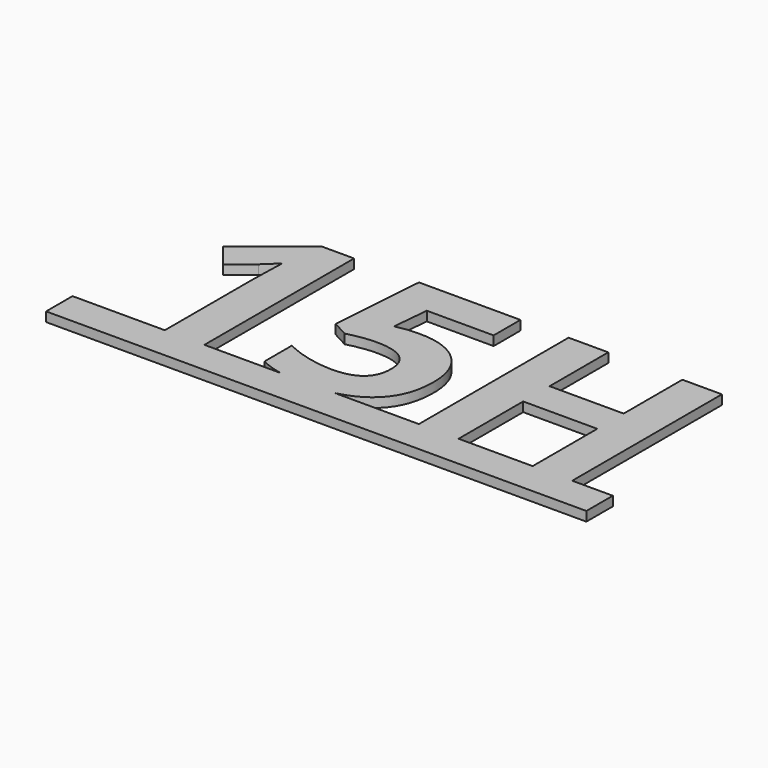
from build123d import *

# Parameters (mm, degrees)
F1_DEPTH = 50.8


# Not quite as in the source:
# - a feature names something its author has since deleted; it is built from what else it names


with BuildPart() as f1:
    # F0 (on Top) → F1 (new body)
    with BuildSketch(Plane.XY):
        with BuildLine():
            Line((-283.7137092352, 0), (-283.7137092352, -177.8))
            Line((-283.7137092352, -177.8), (2624.9390685426, -177.8))
            Line((2624.9390685426, -177.8), (2624.9390685426, 0))
            Line((2624.9390685426, 0), (2406.4373324315, 0))
            Line((2406.4373324315, 0), (2193.4477490981, 0))
            Line((2193.4477490981, 0), (1794.5883740981, 0))
            Line((1794.5883740981, 0), (1580.9373324315, 0))
            Line((1580.9373324315, 0), (1126.7145519045, 0))
            add(Edge.make_bspline(
                [(1126.7145519045, 0), (1064.7611763958, -13.890625), (989.1526102093, -13.890625)],
                knots=[0.6094332671, 0.6094332671, 0.6094332671, 1, 1, 1], degree=2))
            add(Edge.make_bspline(
                [(989.1526102093, -13.890625), (904.1900533476, -13.890625), (835.8175141984, 0)],
                knots=[0, 0, 0, 0.5050353738, 0.5050353738, 0.5050353738], degree=2))
            Line((835.8175141984, 0), (426.2515685426, 0))
            Line((426.2515685426, 0), (213.2619852093, 0))
            Line((213.2619852093, 0), (-283.7137092352, 0))
        make_face()
        with BuildLine():
            add(Edge.make_bspline(
                [(835.8175141984, 0), (768.808369802, 13.6136365267), (717.7342074315, 40.5694444444)],
                knots=[0.5050353738, 0.5050353738, 0.5050353738, 1, 1, 1], degree=2))
            Line((835.8175141984, 0), (1126.7145519045, 0))
            add(Edge.make_bspline(
                [(1286.8088602093, 77.1701388889), (1223.3854786806, 21.6746800513), (1126.7145519045, 0)],
                knots=[0, 0, 0, 0.6094332671, 0.6094332671, 0.6094332671], degree=2))
            add(Edge.make_bspline(
                [(1390.8783046537, 336.9027777778), (1390.8783046537, 168.2309027778), (1286.8088602093, 77.1701388889)],
                knots=[0, 0, 0, 1, 1, 1], degree=2))
            add(Edge.make_bspline(
                [(1304.3375060426, 561.578125), (1390.8783046537, 479.5572916667), (1390.8783046537, 336.9027777778)],
                knots=[0, 0, 0, 1, 1, 1], degree=2))
            add(Edge.make_bspline(
                [(1071.8349018759, 643.5989583333), (1217.7967074315, 643.5989583333), (1304.3375060426, 561.578125)],
                knots=[0, 0, 0, 1, 1, 1], degree=2))
            add(Edge.make_bspline(
                [(967.7654574315, 633.8975694444), (1009.8783046537, 643.5989583333), (1071.8349018759, 643.5989583333)],
                knots=[0, 0, 0, 1, 1, 1], degree=2))
            Line((967.7654574315, 633.8975694444), (943.7324713204, 629.046875))
            Line((943.7324713204, 629.046875), (962.2533046537, 826.8229166667))
            Line((962.2533046537, 826.8229166667), (1321.8661518759, 826.8229166667))
            Line((1321.8661518759, 826.8229166667), (1321.8661518759, 1007.4010416667))
            Line((1321.8661518759, 1007.4010416667), (775.5015685426, 1007.4010416667))
            Line((775.5015685426, 1007.4010416667), (737.5779574315, 494.109375))
            Line((737.5779574315, 494.109375), (822.4651102093, 448.46875))
            add(Edge.make_bspline(
                [(894.1230963204, 464.1232638889), (850.0258740981, 456.8472222222), (822.4651102093, 448.46875)],
                knots=[0, 0, 0, 1, 1, 1], degree=2))
            add(Edge.make_bspline(
                [(974.6005268759, 471.3993055556), (938.2203185426, 471.3993055556), (894.1230963204, 464.1232638889)],
                knots=[0, 0, 0, 1, 1, 1], degree=2))
            add(Edge.make_bspline(
                [(1176.5658046537, 319.0434027778), (1176.5658046537, 471.3993055556), (974.6005268759, 471.3993055556)],
                knots=[0, 0, 0, 1, 1, 1], degree=2))
            add(Edge.make_bspline(
                [(981.4355963204, 159.1909722222), (1176.5658046537, 159.1909722222), (1176.5658046537, 319.0434027778)],
                knots=[0, 0, 0, 1, 1, 1], degree=2))
            add(Edge.make_bspline(
                [(844.4034782648, 177.4913194444), (916.8331657648, 159.1909722222), (981.4355963204, 159.1909722222)],
                knots=[0, 0, 0, 1, 1, 1], degree=2))
            add(Edge.make_bspline(
                [(717.7342074315, 224.6753472222), (771.9737907648, 195.7916666667), (844.4034782648, 177.4913194444)],
                knots=[0, 0, 0, 1, 1, 1], degree=2))
            Line((717.7342074315, 224.6753472222), (717.7342074315, 40.5694444444))
        make_face()
        Polygon((2193.4477490981, 0), (2406.4373324315, 0), (2406.4373324315, 1007.4010416667), (2193.4477490981, 1007.4010416667), (2193.4477490981, 612.5104166667), (1794.5883740981, 612.5104166667), (1794.5883740981, 1007.4010416667), (1580.9373324315, 1007.4010416667), (1580.9373324315, 0), (1794.5883740981, 0), (1794.5883740981, 434.7986111111), (2193.4477490981, 434.7986111111), align=None)
        with BuildLine():
            Line((213.2619852093, 582.9652777778), (213.2619852093, 0))
            Line((213.2619852093, 0), (426.2515685426, 0))
            Line((426.2515685426, 0), (426.2515685426, 1007.4010416667))
            Line((426.2515685426, 1007.4010416667), (251.1855963204, 1007.4010416667))
            Line((251.1855963204, 1007.4010416667), (-73.3699592352, 748.9913194444))
            Line((-73.3699592352, 748.9913194444), (29.3765685426, 620.8888888889))
            Line((29.3765685426, 620.8888888889), (145.1317768759, 713.9340277778))
            add(Edge.make_bspline(
                [(218.774137987, 783.3871527778), (165.8574713204, 730.4704861111), (145.1317768759, 713.9340277778)],
                knots=[0, 0, 0, 1, 1, 1], degree=2))
            Line((218.774137987, 783.3871527778), (215.4668463204, 678.65625))
            Line((215.4668463204, 678.65625), (213.2619852093, 582.9652777778))
        make_face()
        with BuildLine():
            Line((1126.7145519045, 0), (835.8175141984, 0))
            add(Edge.make_bspline(
                [(989.1526102093, -13.890625), (904.1900533476, -13.890625), (835.8175141984, 0)],
                knots=[0, 0, 0, 0.5050353738, 0.5050353738, 0.5050353738], degree=2))
            add(Edge.make_bspline(
                [(1126.7145519045, 0), (1064.7611763958, -13.890625), (989.1526102093, -13.890625)],
                knots=[0.6094332671, 0.6094332671, 0.6094332671, 1, 1, 1], degree=2))
        make_face()
    extrude(amount=F1_DEPTH)


solid = f1.part
